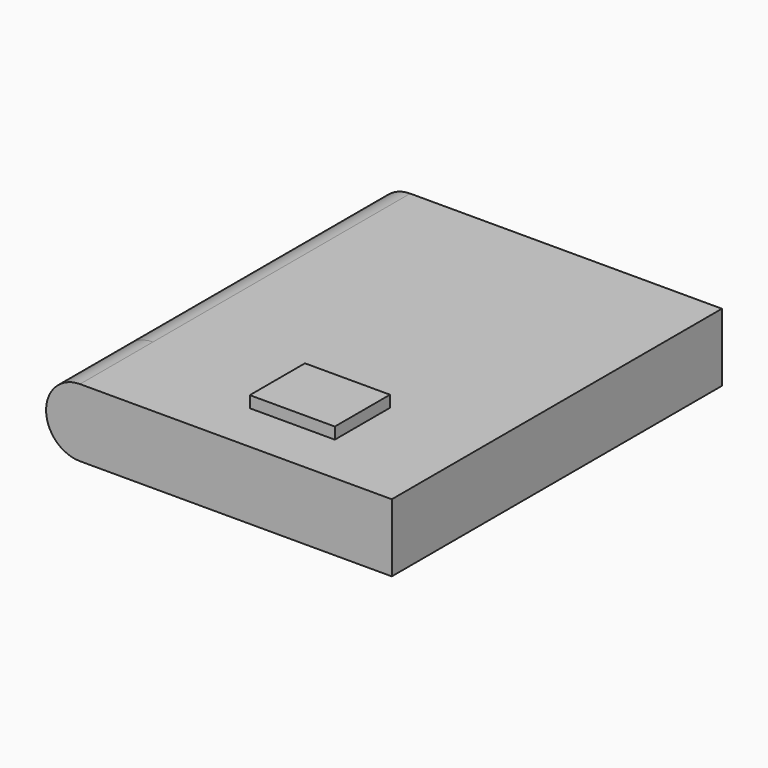
from build123d import *

# Parameters (mm, degrees)
F0_W     = 51.7186559737
F0_H     = 32.6044745743
F1_DEPTH = 10.16
F2_DEPTH = 15.494
F4_R     = 5.08
F5_R     = 5.07999
F6_DEPTH = 13.6398
F7_W     = 12.719899416
F7_H     = 10.316294618
F8_DEPTH = 1.7272


# Not quite as in the source:
# - a fillet or chamfer is up to 0.001 mm smaller than in the source, because OpenCascade refuses the exact size


with BuildPart() as f1:
    # F0 (on Top) → F1 (new body)
    with BuildSketch(Plane.XY):
        with Locations((25.8593279868, 16.3022372872)):
            Rectangle(F0_W, F0_H)
    extrude(amount=F1_DEPTH)

    # F2 (add): a face of the model
    f2_faces = [f1.faces().sort_by_distance(p)[0] for p in [
        (25.8593279868, 0, 5.08),
    ]]
    extrude(f2_faces, amount=F2_DEPTH)

    # F4
    f4_edges = [f1.edges().sort_by_distance(p)[0] for p in [
        (0, 8.555237, 10.16),
    ]]
    fillet(f4_edges, radius=F4_R)

    # F5 (radius 5.08 in the source; OpenCascade refuses exactly that, so slightly less here)
    f5_edges = [f1.edges().sort_by_distance(p)[0] for p in [
        (0, 8.555237, 0),
    ]]
    fillet(f5_edges, radius=F5_R)

    # F6 (add): a face of the model
    f6_faces = [f1.faces().sort_by_distance(p)[0] for p in [
        (26.3917193742, -15.494, 5.0799998568),
    ]]
    extrude(f6_faces, amount=F6_DEPTH)

    # F7 (on face) → F8 (join)
    with BuildSketch(Plane.XY.offset(10.16)):
        with Locations((30.7424403727, -16.3579261862)):
            Rectangle(F7_W, F7_H)
    extrude(amount=F8_DEPTH)


solid = f1.part
